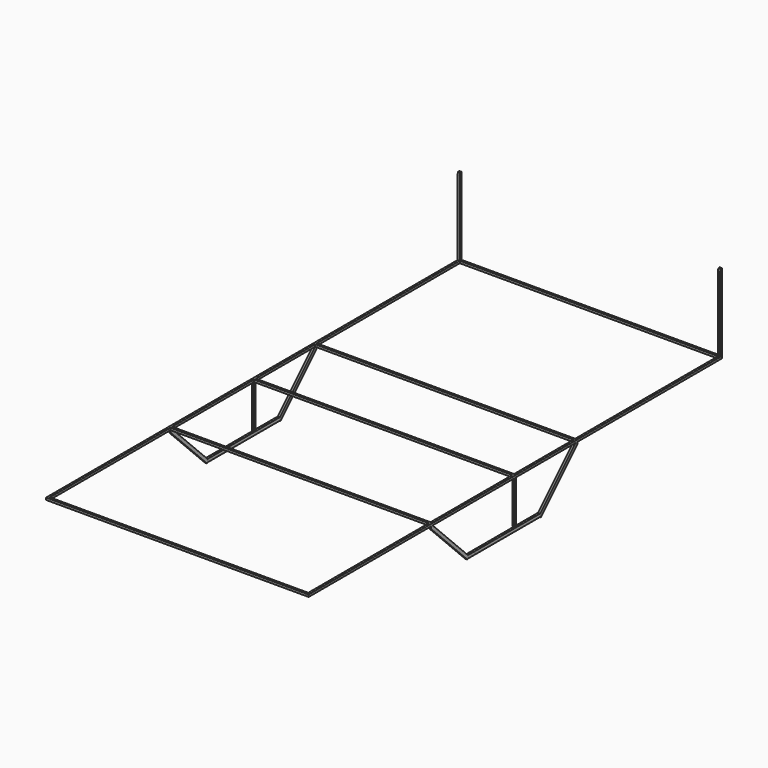
from build123d import *

# Parameters (mm, degrees)
F0_W           = 12.7
F0_H           = 12.7
F1_DEPTH       = 3048
F2_W           = 12.7
F2_H           = 12.7
F3_DEPTH       = 1524
F5_DEPTH       = 1539.24
F6_W           = 12.7
F6_H           = 12.7
F7_DEPTH       = 254
F8_W           = 12.7
F8_H           = 12.7
F9_DEPTH       = 1549.4
F10_W          = 12.7
F10_H          = 12.7
F11_DEPTH      = 1549.4
F12_W          = 12.7
F12_H          = 12.6888751984
F13_DEPTH      = 12.7
F12_W_2        = 12.6959085464
F12_H_2        = 12.7
F14_T1_DEPTH   = 78.0207478943
F14_2_T1_DEPTH = 78.0166564408
F15_SIZE2      = 12.69999
F15_SIZE       = 12.69999
F15_2_SIZE2    = 12.69999
F15_2_SIZE     = 12.69999
F16_DEPTH      = 381
F17_SIZE2      = 12.7
F17_SIZE       = 12.7
F17_2_SIZE2    = 12.7
F17_2_SIZE     = 12.7
F18_DEPTH      = 482.6
F19_DEPTH      = 381
F20_SIZE2      = 12.7
F20_SIZE       = 12.7
F20_2_SIZE2    = 12.7
F20_2_SIZE     = 12.7
F21_DEPTH      = 127
F22_W          = 12.7
F22_H          = 12.7
F23_DEPTH      = 457.2
F24_SIZE2      = 2.239352655
F24_SIZE       = 12.7
F25_SIZE2      = 12.7
F25_SIZE       = 2.286


# Not quite as in the source:
# - a fillet or chamfer that OpenCascade refuses, or shapes differently, is made with other operations: its cross-section is extruded or revolved along the edge and cut away or added
# - a fillet or chamfer is up to 0.001 mm smaller than in the source, because OpenCascade refuses the exact size


with BuildPart() as f1:
    # F0 (on Front) → F1 (new body)
    with BuildSketch(Plane.XZ):
        with Locations((1480.6543715816, -6.35)):
            Rectangle(F0_W, F0_H)
    extrude(amount=F1_DEPTH)


with BuildPart() as f1b:
    # F0 (on Front) → F1, piece 2 (new body)
    with BuildSketch(Plane.XZ):
        with Locations((-56.0456284184, -6.35)):
            Rectangle(F0_W, F0_H)
    extrude(amount=F1_DEPTH)


with BuildPart() as f3:
    # F2 (on face) → F3 (new body)
    with BuildSketch(Plane(origin=(1474.3043715816, 0, 0), x_dir=(0, -1, 0), z_dir=(-1, 0, 0))):
        with Locations((6.35, -6.35)):
            Rectangle(F2_W, F2_H)
    extrude(amount=F3_DEPTH)


with BuildPart() as f3b:
    # F2 (on face) → F3, piece 2 (new body)
    with BuildSketch(Plane(origin=(1474.3043715816, 0, 0), x_dir=(0, -1, 0), z_dir=(-1, 0, 0))):
        with Locations((3041.65, -6.35)):
            Rectangle(F2_W, F2_H)
    extrude(amount=F3_DEPTH)


with BuildPart() as f5:
    # F4 (on face) → F5 (new body)
    with BuildSketch(Plane.YZ.offset(1487.0043715816)):
        Polygon((-1530.35, -0.0233579591), (-1530.35, -12.7), (-1524, -12.7), (-1517.65, -12.7), (-1517.65, -0.0233579591), align=None)
    extrude(amount=-F5_DEPTH)


with BuildPart() as f7:
    # F6 (on face) → F7 (new body)
    with BuildSketch(Plane(origin=(0, 0, -12.7), x_dir=(1, 0, 0), z_dir=(0, 0, -1))):
        with Locations((1480.6543715816, 1524.0000082016)):
            Rectangle(F6_W, F6_H)
    extrude(amount=F7_DEPTH)


with BuildPart() as f7b:
    # F6 (on face) → F7, piece 2 (new body)
    with BuildSketch(Plane(origin=(0, 0, -12.7), x_dir=(1, 0, 0), z_dir=(0, 0, -1))):
        with Locations((-56.0456471682, 1524.0001274109)):
            Rectangle(F6_W, F6_H)
    extrude(amount=F7_DEPTH)


with BuildPart() as f9:
    # F8 (on face) → F9 (new body)
    with BuildSketch(Plane.YZ.offset(1487.0043715816)):
        with Locations((-2139.95, -6.35)):
            Rectangle(F8_W, F8_H)
    extrude(amount=-F9_DEPTH)


with BuildPart() as f11:
    # F10 (on face) → F11 (new body)
    with BuildSketch(Plane(origin=(-62.3956284184, 0, 0), x_dir=(0, -1, 0), z_dir=(-1, 0, 0))):
        with Locations((1073.15, -6.35)):
            Rectangle(F10_W, F10_H)
    extrude(amount=-F11_DEPTH)


with BuildPart() as f13:
    # F12 (on face) → F13 (new body)
    with BuildSketch(Plane(origin=(0, 0, -12.7), x_dir=(1, 0, 0), z_dir=(0, 0, -1))):
        with Locations((-56.0456284184, 2139.9773359299)):
            Rectangle(F12_W, F12_H)
    extrude(amount=F13_DEPTH)

    # F14: chamfer of 12.7 on 1 edges, made by hand

    # F14_s2 → F14_t1 (cut)
    with BuildSketch(Plane.YZ.offset(-95.0560023656)):
        Polygon((-2133.6328983307, -12.7), (-2146.3328983307, -25.4), (-2133.6328983307, -25.4), align=None)
    extrude(amount=F14_T1_DEPTH, mode=Mode.SUBTRACT)


with BuildPart() as f13b:
    # F12 (on face) → F13, piece 2 (new body)
    with BuildSketch(Plane(origin=(0, 0, -12.7), x_dir=(1, 0, 0), z_dir=(0, 0, -1))):
        with Locations((1480.6722998619, 2139.9773359299)):
            Rectangle(F12_W_2, F12_H)
    extrude(amount=F13_DEPTH)

    # F14#2: chamfer of 12.7 on 1 edges, made by hand

    # F14_2_s2 → F14_2_t1 (cut)
    with BuildSketch(Plane.YZ.offset(1441.6639716415)):
        Polygon((-2133.6328983307, -12.7), (-2146.3328983307, -25.4), (-2133.6328983307, -25.4), align=None)
    extrude(amount=F14_2_T1_DEPTH, mode=Mode.SUBTRACT)


with BuildPart() as f13c:
    # F12 (on face) → F13, piece 3 (new body)
    with BuildSketch(Plane(origin=(0, 0, -12.7), x_dir=(1, 0, 0), z_dir=(0, 0, -1))):
        with Locations((1480.6743455887, 1072.9938341141)):
            Rectangle(F12_W, F12_H_2)
    extrude(amount=F13_DEPTH)

    # F15 (size 12.7 and 12.7 in the source; OpenCascade refuses exactly that, so slightly less here)
    f15_edges = [f13c.edges().sort_by_distance(p)[0] for p in [
        (1480.674346, -1079.343834, -25.4),
    ]]
    chamfer(f15_edges, length=F15_SIZE, length2=F15_SIZE2)


with BuildPart() as f13d:
    # F12 (on face) → F13, piece 4 (new body)
    with BuildSketch(Plane(origin=(0, 0, -12.7), x_dir=(1, 0, 0), z_dir=(0, 0, -1))):
        with Locations((-56.0456284184, 1073.0461669922)):
            Rectangle(F12_W, F12_H_2)
    extrude(amount=F13_DEPTH)

    # F15#2 (size 12.7 and 12.7 in the source; OpenCascade refuses exactly that, so slightly less here)
    f15_2_edges = [f13d.edges().sort_by_distance(p)[0] for p in [
        (-56.045628, -1079.396167, -25.4),
    ]]
    chamfer(f15_2_edges, length=F15_2_SIZE, length2=F15_2_SIZE2)


with BuildPart() as f16:
    # F16 (new): a face of the model
    f16_faces = [f13c.part.faces().sort_by_distance(p)[0] for p in [
        (1480.6743455887, -1072.9938391141, -19.050005),
    ]]
    extrude(f16_faces, amount=F16_DEPTH)

    # F17
    f17_edges = [f16.edges().sort_by_distance(p)[0] for p in [
        (1480.674346, -1348.751518, -282.107694),
    ]]
    chamfer(f17_edges, length=F17_SIZE, length2=F17_SIZE2)


with BuildPart() as f16b:
    # F16#2 (new): a face of the model
    f16_2_faces = [f13d.part.faces().sort_by_distance(p)[0] for p in [
        (-56.0456284184, -1073.0461719922, -19.050005),
    ]]
    extrude(f16_2_faces, amount=F16_DEPTH)

    # F17#2
    f17_2_edges = [f16b.edges().sort_by_distance(p)[0] for p in [
        (-56.045628, -1348.803851, -282.107694),
    ]]
    chamfer(f17_2_edges, length=F17_2_SIZE, length2=F17_2_SIZE2)


with BuildPart() as f18:
    # F18 (new): a face of the model
    f18_faces = [f16b.part.faces().sort_by_distance(p)[0] for p in [
        (-56.0456284184, -1339.8235945032, -282.1076936321),
    ]]
    extrude(f18_faces, amount=F18_DEPTH)


with BuildPart() as f18b:
    # F18#2 (new): a face of the model
    f18_2_faces = [f16.part.faces().sort_by_distance(p)[0] for p in [
        (1480.6743455887, -1339.7712616251, -282.1076936321),
    ]]
    extrude(f18_2_faces, amount=F18_DEPTH)


with BuildPart() as f19:
    # F19 (new): a face of the model
    f19_faces = [f13.part.faces().sort_by_distance(p)[0] for p in [
        (-56.0456284184, -2139.9773359299, -19.0444375992),
    ]]
    extrude(f19_faces, amount=F19_DEPTH)

    # F20
    f20_edges = [f19.edges().sort_by_distance(p)[0] for p in [
        (-56.045628, -1864.225215, -282.107684),
    ]]
    chamfer(f20_edges, length=F20_SIZE, length2=F20_SIZE2)


with BuildPart() as f19b:
    # F19#2 (new): a face of the model
    f19_2_faces = [f13b.part.faces().sort_by_distance(p)[0] for p in [
        (1480.6722998619, -2139.9773359299, -19.0444375992),
    ]]
    extrude(f19_2_faces, amount=F19_DEPTH)

    # F20#2
    f20_2_edges = [f19b.edges().sort_by_distance(p)[0] for p in [
        (1480.6723, -1864.225215, -282.107684),
    ]]
    chamfer(f20_2_edges, length=F20_2_SIZE, length2=F20_2_SIZE2)


with BuildPart() as f21:
    # F21 (new): a face of the model
    f21_faces = [f19.part.faces().sort_by_distance(p)[0] for p in [
        (-56.0456284184, -1873.2054708197, -282.1076836321),
    ]]
    extrude(f21_faces, amount=F21_DEPTH)


with BuildPart() as f21b:
    # F21#2 (new): a face of the model
    f21_2_faces = [f19b.part.faces().sort_by_distance(p)[0] for p in [
        (1480.6722998619, -1873.2054708197, -282.1076836321),
    ]]
    extrude(f21_2_faces, amount=F21_DEPTH)


with BuildPart() as f23:
    # F22 (on face) → F23 (new body)
    with BuildSketch(Plane.XY):
        with Locations((-56.0456284184, -6.35)):
            Rectangle(F22_W, F22_H)
    extrude(amount=F23_DEPTH)

    # F25
    f25_edges = [f23.edges().sort_by_distance(p)[0] for p in [
        (-56.045628, -12.7, 457.2),
    ]]
    f25_side = f23.faces().sort_by_distance((-56.045628, -6.35, 457.2))[0]
    chamfer(f25_edges, length=F25_SIZE, length2=F25_SIZE2, reference=f25_side)


with BuildPart() as f23b:
    # F22 (on face) → F23, piece 2 (new body)
    with BuildSketch(Plane.XY):
        with Locations((1480.6544376373, -6.35)):
            Rectangle(F22_W, F22_H)
    extrude(amount=F23_DEPTH)

    # F24
    f24_edges = [f23b.edges().sort_by_distance(p)[0] for p in [
        (1480.654438, -12.7, 457.2),
    ]]
    f24_side = f23b.faces().sort_by_distance((1480.654438, -12.7, 228.6))[0]
    chamfer(f24_edges, length=F24_SIZE, length2=F24_SIZE2, reference=f24_side)


solid = Compound([f1.part, f1b.part, f3.part, f3b.part, f5.part, f7.part, f7b.part, f9.part, f11.part, f13.part, f13b.part, f13c.part, f13d.part, f16.part, f16b.part, f18.part, f18b.part, f19.part, f19b.part, f21.part, f21b.part, f23.part, f23b.part])
